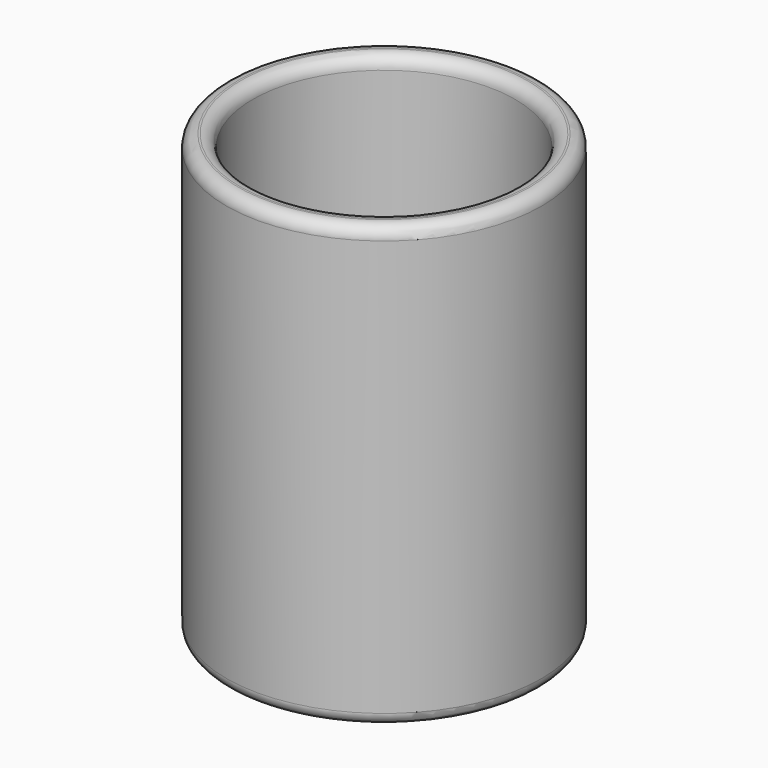
from build123d import *

# Parameters (mm, degrees)
F0_R     = 8.95
F0_R_2   = 7.45
F1_DEPTH = 25
F2_START = 12
F0_R_3   = 5.95
F2_DEPTH = 1
F3_R     = 0.7
F4_R     = 0.49999


# Not quite as in the source:
# - a fillet or chamfer is up to 0.001 mm smaller than in the source, because OpenCascade refuses the exact size


with BuildPart() as f1:
    # F0 (on Top) → F1 (new body)
    with BuildSketch(Plane.XY):
        Circle(F0_R)
        Circle(F0_R_2, mode=Mode.SUBTRACT)
    extrude(amount=F1_DEPTH)

    # F0 (on Top) → F2 (join)
    with BuildSketch(Plane.XY.offset(F2_START)):
        Circle(F0_R_2)
        Circle(F0_R_3, mode=Mode.SUBTRACT)
    extrude(amount=F2_DEPTH)

    # F3
    f3_edges = [f1.edges().sort_by_distance(p)[0] for p in [
        (-8.95, 0, 25),
        (-7.45, 0, 25),
        (-8.95, 0, 0),
        (-7.45, 0, 0),
    ]]
    fillet(f3_edges, radius=F3_R)

    # F4 (radius 0.5 in the source; OpenCascade refuses exactly that, so slightly less here)
    f4_edges = [f1.edges().sort_by_distance(p)[0] for p in [
        (5.95, 0, 12.5),
        (-5.95, 0, 12),
        (-5.95, 0, 13),
    ]]
    fillet(f4_edges, radius=F4_R)


solid = f1.part
